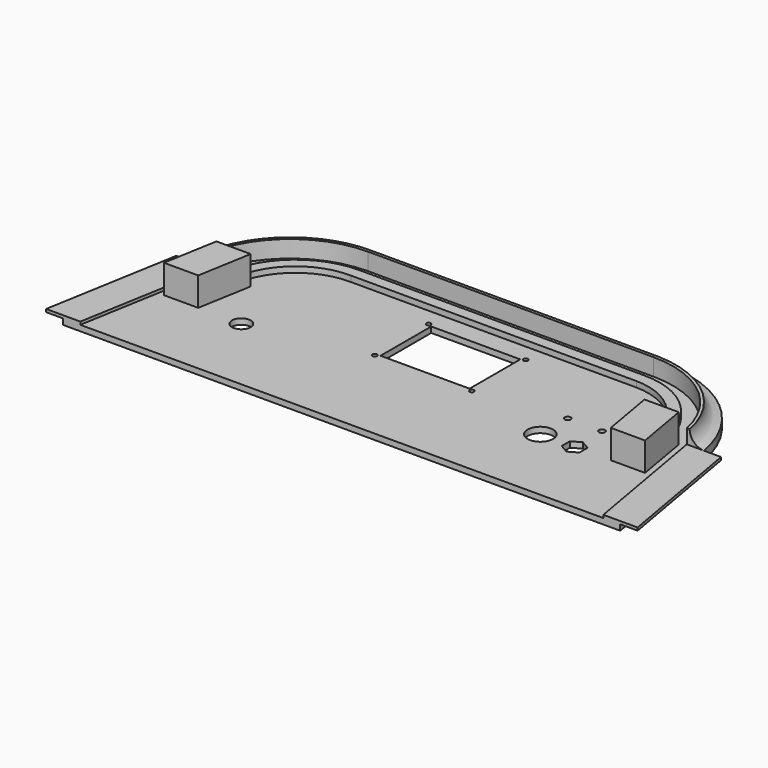
from build123d import *

# Parameters (mm, degrees)
F1_DEPTH  = 5
F3_DEPTH  = 15
F8_DEPTH  = 2.5
F9_W      = 78
F9_H      = 55.5
F9_R      = 2
F10_DEPTH = 25
F11_R     = 11.15
F11_R_2   = 2.65
F12_DEPTH = 25
F13_R     = 8.15
F14_DEPTH = 25
F16_DEPTH = 25
F17_W     = 10
F17_H     = 5
F17_R     = 2.5


with BuildPart() as f1:
    # F0 (on Top) → F1 (new body)
    with BuildSketch(Plane.XY):
        with BuildLine():
            Line((20.3815252042, 117.1415335559), (0, 0))
            Line((0, 0), (487.8028212909, 0))
            Line((487.8028212909, 0), (467.4212960867, 117.1415335559))
            ThreePointArc((467.4212960867, 117.1415335559), (433.2669551721, 176.5315404118), (368.9014106455, 200))
            Line((368.9014106455, 200), (118.9014106455, 200))
            ThreePointArc((118.9014106455, 200), (54.5358661189, 176.5315404118), (20.3815252042, 117.1415335559))
        make_face()
    extrude(amount=-F1_DEPTH)

    # F2 (on face) → F3 (join)
    with BuildSketch(Plane.XY):
        with BuildLine():
            Line((368.9014106455, 200), (118.9014106455, 200))
            ThreePointArc((118.9014106455, 200), (54.5358661189, 176.5315404118), (20.3815252042, 117.1415335559))
            Line((20.3815252042, 117.1415335559), (35.3815252042, 117.1415335559))
            ThreePointArc((35.3815252042, 117.1415335559), (65.0954102081, 165.8969986874), (118.9014106455, 185))
            Line((118.9014106455, 185), (368.9014106455, 185))
            ThreePointArc((368.9014106455, 185), (422.7074110828, 165.8969986874), (452.4212960867, 117.1415335559))
            Line((452.4212960867, 117.1415335559), (467.4212960867, 117.1415335559))
            ThreePointArc((467.4212960867, 117.1415335559), (433.2669551721, 176.5315404118), (368.9014106455, 200))
        make_face()
    extrude(amount=F3_DEPTH)

    # F6: sweep along a path in F5
    with BuildLine(Plane.XY.offset(15)) as f6_path:
        ThreePointArc((20.3815252042, 117.1415335559), (54.5358661189, 176.5315404118), (118.9014106455, 200))
        Line((118.9014106455, 200), (368.9014106455, 200))
        ThreePointArc((368.9014106455, 200), (433.2669551721, 176.5315404118), (467.4212960867, 117.1415335559))
    # F4 (on face) → F6 (sweep, cut)
    with BuildSketch(Plane.XZ.offset(-117.1415335559)):
        with BuildLine():
            ThreePointArc((20.3815252042, 2.5), (29.2203599691, 6.1611652352), (32.8815252042, 15))
            Line((32.8815252042, 15), (20.3815252042, 15))
            Line((20.3815252042, 15), (20.3815252042, 2.5))
        make_face()
    sweep(path=f6_path.line, mode=Mode.SUBTRACT)

    # F7 (on face) → F8 (join)
    with BuildSketch(Plane.XY):
        Polygon((-15, 0), (0, 0), (20.3815252042, 117.1415335559), (5.3815252042, 117.1415335559), align=None)
        Polygon((0, 0), (15, 0), (35.3815252042, 117.1415335559), (20.3815252042, 117.1415335559), align=None)
        Polygon((452.4212960867, 117.1415335559), (473.0281739523, 0), (487.8028212909, 0), (467.4212960867, 117.1415335559), align=None)
        Polygon((467.4212960867, 117.1415335559), (487.8028212909, 0), (503.0281739523, 0), (482.4212960867, 117.1415335559), align=None)
    extrude(amount=F8_DEPTH)

    # F9 (on face) → F10 (cut)
    with BuildSketch(Plane(origin=(0, 0, -5), x_dir=(1, 0, 0), z_dir=(0, 0, -1))):
        with Locations((242.9, -120.25)):
            Rectangle(F9_W, F9_H)
        with Locations((200.2686832967, -149.75)):
            Circle(F9_R)
        with Locations((200.2686832967, -90.75)):
            Circle(F9_R)
        with Locations((285.2686832967, -90.75)):
            Circle(F9_R)
        with Locations((285.2686832967, -149.75)):
            Circle(F9_R)
    extrude(amount=-F10_DEPTH, mode=Mode.SUBTRACT)

    # F11 (on face) → F12 (cut)
    with BuildSketch(Plane(origin=(0, 0, -5), x_dir=(1, 0, 0), z_dir=(0, 0, -1))):
        Polygon((391.9, -78.9489291724), (399.65, -74.4744645862), (399.65, -65.5255354138), (391.9, -61.0510708276), (384.15, -65.5255354138), (384.15, -74.4744645862), align=None)
        with Locations((361.9, -70)):
            Circle(F11_R)
        with Locations((361.9, -100)):
            Circle(F11_R_2)
        with Locations((391.9, -100)):
            Circle(F11_R_2)
    extrude(amount=-F12_DEPTH, mode=Mode.SUBTRACT)

    # F13 (on face) → F14 (cut)
    with BuildSketch(Plane.XY):
        with Locations((100, 70)):
            Circle(F13_R)
    extrude(amount=-F14_DEPTH, mode=Mode.SUBTRACT)

    # F15 (on face) → F16 (join)
    with BuildSketch(Plane.XY):
        Polygon((40.456642758, 117.1415335559), (32.2544592526, 70), (62.2544592526, 70), (70.456642758, 117.1415335559), align=None)
        Polygon((415.343357242, 117.1415335559), (423.5455407474, 70), (453.5455407474, 70), (445.343357242, 117.1415335559), align=None)
    extrude(amount=F16_DEPTH)

    # F19: sweep along a path in F18
    with BuildLine(Plane.XY) as f19_path:
        ThreePointArc((55.456642758, 117.1415335559), (77.6120171917, 155.0538221629), (118.9014106455, 170))
        Line((118.9014106455, 170), (368.9014106455, 170))
        ThreePointArc((368.9014106455, 170), (409.4264963221, 154.9669307173), (430.343357242, 117.1415335559))
        Line((430.343357242, 117.1415335559), (431.8368507266, 107.2536886334))
    # F17 (on face) → F19 (sweep)
    with BuildSketch(Plane(origin=(0, 117.1415335559, 0), x_dir=(-1, 0, 0), z_dir=(0, 1, 0))):
        with Locations((-55.456642758, 2.5)):
            Rectangle(F17_W, F17_H)
        with Locations((-55.456642758, -4)):
            Circle(F17_R)
    sweep(path=f19_path.line)


solid = f1.part
